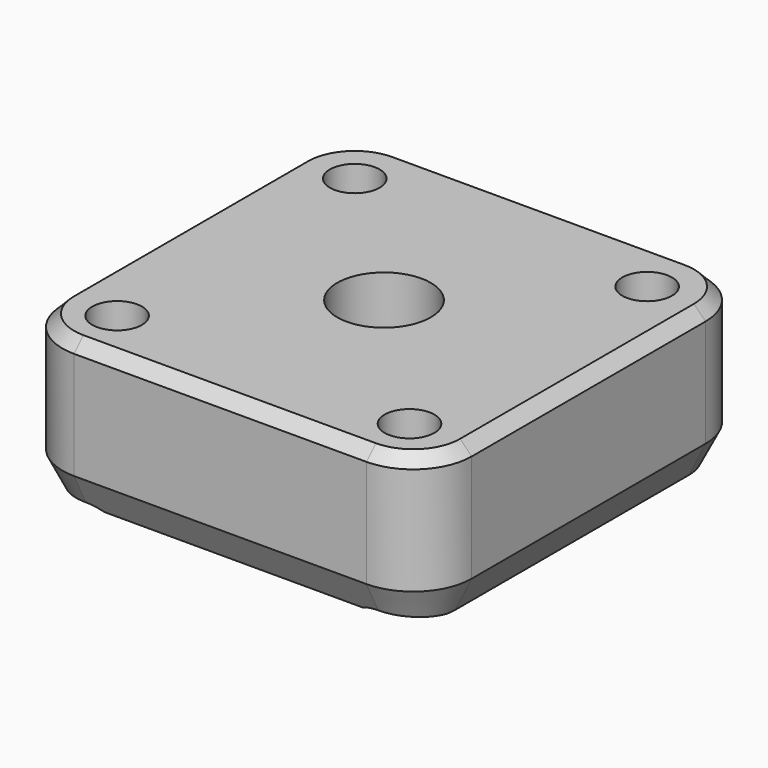
from build123d import *

# Parameters (mm, degrees)
F0_W         = 35
F0_H         = 35
F1_DEPTH     = 6.5
F2_R         = 2.125
F3_DEPTH     = 13.001
F4_R         = 5
F5_T1_DEPTH  = 25
F5_T3_DEPTH  = 25
F5_T12_ANGLE = 90
F5_T14_ANGLE = 90
F5_T16_ANGLE = 90
F5_T18_ANGLE = 90
F6_R         = 4
F7_DEPTH     = 13.001
F8_SIZE      = 1


# Not quite as in the source:
# - a fillet or chamfer that OpenCascade refuses, or shapes differently, is made with other operations: its cross-section is extruded or revolved along the edge and cut away or added


with BuildPart() as f1:
    # F0 (on Top) → F1 (new body, symmetric)
    with BuildSketch(Plane.XY):
        Rectangle(F0_W, F0_H)
    extrude(amount=F1_DEPTH, both=True)

    # F2 (on face) → F3 (cut, through all)
    with BuildSketch(Plane.XY.offset(6.5)):
        with Locations((-12.5, -12.9)):
            Circle(F2_R)
        with Locations((-12.5, 12.5)):
            Circle(F2_R)
        with Locations((12.5, 12.5)):
            Circle(F2_R)
        with Locations((12.5, -12.9)):
            Circle(F2_R)
    extrude(amount=-F3_DEPTH, mode=Mode.SUBTRACT)

    # F4
    f4_edges = [f1.edges().sort_by_distance(p)[0] for p in [
        (-17.5, 17.5, 0),
        (17.5, 17.5, 0),
        (17.5, -17.5, 0),
        (-17.5, -17.5, 0),
    ]]
    fillet(f4_edges, radius=F4_R)

    # F5: chamfer of 1.4 x 2.8 on 12 edges, made by hand

    # F5_s2 → F5_t1 (cut)
    with BuildSketch(Plane.XZ.offset(-12.5)):
        Polygon((17.5, -3.7), (16.1, -6.5), (17.5, -6.5), align=None)
        Polygon((-16.1, -6.5), (-17.5, -3.7), (-17.5, -6.5), align=None)
    extrude(amount=F5_T1_DEPTH, mode=Mode.SUBTRACT)

    # F5_s4 → F5_t3 (cut)
    with BuildSketch(Plane.YZ.offset(-12.5)):
        Polygon((-16.1, -6.5), (-17.5, -3.7), (-17.5, -6.5), align=None)
        Polygon((16.1, -6.5), (17.5, -3.7), (17.5, -6.5), align=None)
    extrude(amount=F5_T3_DEPTH, mode=Mode.SUBTRACT)

    # F5_s5 → F5_t6 (revolve, cut)
    with BuildSketch(Plane.XZ.offset(12.9)):
        Polygon((-8.975, -6.5), (-10.375, -3.7), (-10.375, -6.5), align=None)
    revolve(axis=Axis((-12.5, -12.9, -6.5), (0, 0, 1)), mode=Mode.SUBTRACT)

    # F5_s7 → F5_t8 (revolve, cut)
    with BuildSketch(Plane.XZ.offset(12.9)):
        Polygon((16.025, -6.5), (14.625, -3.7), (14.625, -6.5), align=None)
    revolve(axis=Axis((12.5, -12.9, -6.5), (0, 0, 1)), mode=Mode.SUBTRACT)

    # F5_s9 → F5_t10 (revolve, cut)
    with BuildSketch(Plane.XZ.offset(-12.5)):
        Polygon((16.025, -6.5), (14.625, -3.7), (14.625, -6.5), align=None)
    revolve(axis=Axis((12.5, 12.5, -6.5), (0, 0, 1)), mode=Mode.SUBTRACT)

    # F5_s11 → F5_t12 (revolve, cut)
    with BuildSketch(Plane.XZ.offset(12.5)):
        Polygon((16.1, -6.5), (17.5, -3.7), (17.5, -6.5), align=None)
    revolve(axis=Axis((12.5, -12.5, -6.5), (0, 0, -1)), revolution_arc=F5_T12_ANGLE, mode=Mode.SUBTRACT)

    # F5_s13 → F5_t14 (revolve, cut)
    with BuildSketch(Plane.XZ.offset(-12.5)):
        Polygon((16.1, -6.5), (17.5, -3.7), (17.5, -6.5), align=None)
    revolve(axis=Axis((12.5, 12.5, -6.5), (0, 0, 1)), revolution_arc=F5_T14_ANGLE, mode=Mode.SUBTRACT)

    # F5_s15 → F5_t16 (revolve, cut)
    with BuildSketch(Plane.YZ.offset(-12.5)):
        Polygon((-16.1, -6.5), (-17.5, -3.7), (-17.5, -6.5), align=None)
    revolve(axis=Axis((-12.5, -12.5, -6.5), (0, 0, -1)), revolution_arc=F5_T16_ANGLE, mode=Mode.SUBTRACT)

    # F5_s17 → F5_t18 (revolve, cut)
    with BuildSketch(Plane.YZ.offset(-12.5)):
        Polygon((16.1, -6.5), (17.5, -3.7), (17.5, -6.5), align=None)
    revolve(axis=Axis((-12.5, 12.5, -6.5), (0, 0, 1)), revolution_arc=F5_T18_ANGLE, mode=Mode.SUBTRACT)

    # F5_s19 → F5_t20 (revolve, cut)
    with BuildSketch(Plane.XZ.offset(-12.5)):
        Polygon((-8.975, -6.5), (-10.375, -3.7), (-10.375, -6.5), align=None)
    revolve(axis=Axis((-12.5, 12.5, -6.5), (0, 0, 1)), mode=Mode.SUBTRACT)

    # F6 (on face) → F7 (cut, through all)
    with BuildSketch(Plane(origin=(0, 0, -6.5), x_dir=(1, 0, 0), z_dir=(0, 0, -1))):
        Circle(F6_R)
    extrude(amount=-F7_DEPTH, mode=Mode.SUBTRACT)

    # F8
    f8_edges = [f1.edges().sort_by_distance(p)[0] for p in [
        (-16.035534, -16.035534, 6.5),
    ]]
    chamfer(f8_edges, length=F8_SIZE)


solid = f1.part
